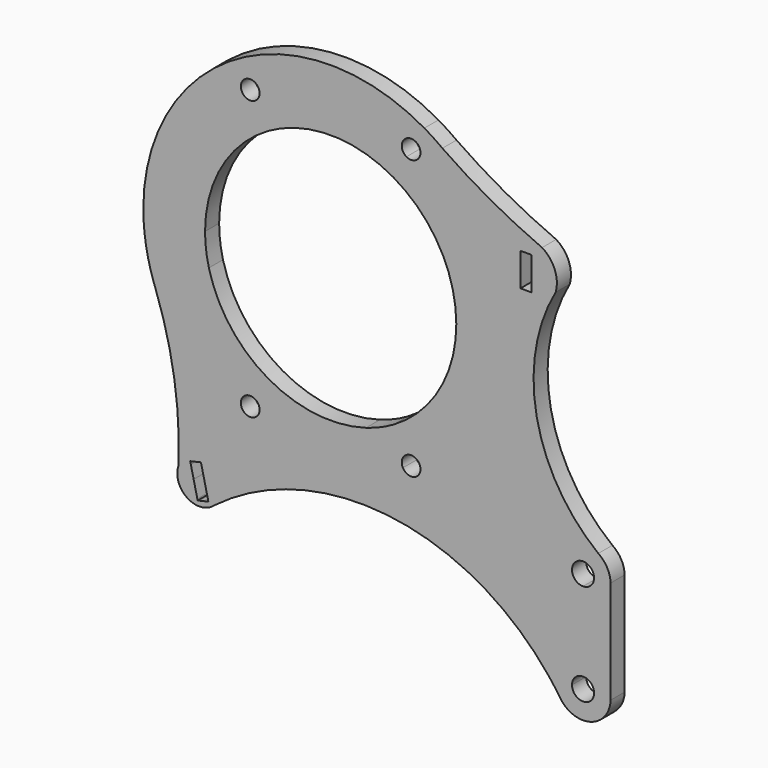
from build123d import *

# Parameters (mm, degrees)
F0_W     = 5
F0_H     = 15
F1_DEPTH = 8


with BuildPart() as f1:
    # F0 (on Front) → F1 (new body)
    with BuildSketch(Plane.XZ):
        with BuildLine():
            ThreePointArc((96.051040545, -74.4952633909), (99.586574451, -75.9597294849), (101.051040545, -79.4952633909))
            Line((101.051040545, -79.4952633909), (108.5446846503, -79.4952633909))
            Line((108.5446846503, -79.4952633909), (108.5446846503, -79.0966947381))
            Line((108.5446846503, -79.0966947381), (108.5446846503, -33.8938320436))
            Line((108.5446846503, -33.8938320436), (108.5446846503, -33.0966947381))
            ThreePointArc((108.5446846503, -33.0966947381), (106.9735378091, -27.4166900782), (102.9745588744, -23.0878192309))
            ThreePointArc((102.9745588744, -23.0878192309), (75.0475031004, 22.3518348869), (83.6459918624, 74.9897356957))
            ThreePointArc((83.6459918624, 74.9897356957), (83.213349074, 83.916829816), (77.4679593625, 90.763046748))
            ThreePointArc((77.4679593625, 90.763046748), (54.2323791008, 102.1278384031), (32.237536797, 115.739509553))
            ThreePointArc((32.237536797, 115.739509553), (46.3985337021, 102.4586914011), (57.1766192186, 86.3110340872))
            ThreePointArc((57.1766192186, 86.3110340872), (64.1749741493, 67.4661239993), (66.5520777255, 47.5047366091))
            ThreePointArc((66.5520777255, 47.5047366091), (55.1642370471, 5.0047366091), (24.0520777255, -26.1074227125))
            ThreePointArc((24.0520777255, -26.1074227125), (11.2153330726, -32.151344654), (-2.4479222745, -35.9758000446))
            Line((-2.4479222745, -35.9758000446), (-2.4479222745, -38.2282986652))
            ThreePointArc((-2.4479222745, -38.2282986652), (43.6638893075, -49.6244865639), (80.5950273587, -79.4952633909))
            Line((80.5950273587, -79.4952633909), (91.051040545, -79.4952633909))
            ThreePointArc((91.051040545, -79.4952633909), (92.5155066391, -75.9597294849), (96.051040545, -74.4952633909))
        make_face()
        with BuildLine():
            ThreePointArc((101.051040545, -33.4952633909), (99.586574451, -37.0307972968), (96.051040545, -38.4952633909))
            ThreePointArc((96.051040545, -38.4952633909), (92.5155066391, -29.9597294849), (101.051040545, -33.4952633909))
        make_face(mode=Mode.SUBTRACT)
        with Locations((70.1775963157, 78.8110340872)):
            Rectangle(F0_W, F0_H, mode=Mode.SUBTRACT)
        with BuildLine():
            Line((108.5446846503, -79.4952633909), (101.051040545, -79.4952633909))
            ThreePointArc((101.051040545, -79.4952633909), (96.051040545, -84.4952633909), (91.051040545, -79.4952633909))
            Line((91.051040545, -79.4952633909), (80.5950273587, -79.4952633909))
            ThreePointArc((80.5950273587, -79.4952633909), (83.0087277773, -82.6464275943), (85.3064858893, -85.8831069432))
            ThreePointArc((85.3064858893, -85.8831069432), (99.1707652013, -91.5996972095), (108.5446846503, -79.8938320436))
            Line((108.5446846503, -79.8938320436), (108.5446846503, -79.4952633909))
        make_face()
        with BuildLine():
            ThreePointArc((-49.4766412308, -47.648732709), (-26.485075504, -40.328623161), (-2.4479222745, -38.2282986652))
            Line((-2.4479222745, -38.2282986652), (-2.4479222745, -35.9758000446))
            ThreePointArc((-2.4479222745, -35.9758000446), (-59.8941418394, -26.7058481061), (-97.9165682257, 17.3429344301))
            ThreePointArc((-97.9165682257, 17.3429344301), (-89.4001229489, -15.7837478144), (-87.5014994409, -49.9349139067))
            ThreePointArc((-87.5014994409, -49.9349139067), (-87.0083312551, -48.7555482085), (-86.3687393855, -47.648732709))
            ThreePointArc((-86.3687393855, -47.648732709), (-82.7667512172, -44.3786510364), (-78.0479222745, -43.1952633909))
            Line((-78.0479222745, -43.1952633909), (-78.0479222745, -42.0817346844))
            Line((-78.0479222745, -42.0817346844), (-77.7900763305, -43.1985881701))
            ThreePointArc((-77.7900763305, -43.1985881701), (-73.2158097389, -44.4402255016), (-69.7271051635, -47.648732709))
            Line((-69.7271051635, -47.648732709), (-49.4766412308, -47.648732709))
        make_face()
        with BuildLine():
            ThreePointArc((-97.9165682257, 17.3429344301), (-59.8941418394, -26.7058481061), (-2.4479222745, -35.9758000446))
            Line((-2.4479222745, -35.9758000446), (-2.4479222745, -23.7202590034))
            ThreePointArc((-2.4479222745, -23.7202590034), (-27.346314823, -24.9508954014), (-51.2070161773, -17.7320763623))
            ThreePointArc((-51.2070161773, -17.7320763623), (-57.0729222745, -19.3957258332), (-58.5651126184, -13.4838774013))
            ThreePointArc((-58.5651126184, -13.4838774013), (-79.0670356762, 6.8313658317), (-90.0928802269, 33.5047366091))
            Line((-90.0928802269, 33.5047366091), (-102.2870539494, 33.5047366091))
            ThreePointArc((-102.2870539494, 33.5047366091), (-100.6924729992, 26.0376949849), (-98.4342508199, 18.7438735165))
            ThreePointArc((-98.4342508199, 18.7438735165), (-98.1739124224, 18.0439571899), (-97.9165682257, 17.3429344301))
        make_face()
        with BuildLine():
            Line((-2.4479222745, -23.7202590034), (-2.4479222745, -35.9758000446))
            ThreePointArc((-2.4479222745, -35.9758000446), (11.2153330726, -32.151344654), (24.0520777255, -26.1074227125))
            Line((24.0520777255, -26.1074227125), (20.1770777255, -19.3957258332))
            ThreePointArc((20.1770777255, -19.3957258332), (16.8924568739, -19.8038559953), (14.3111716282, -17.7320763623))
            ThreePointArc((14.3111716282, -17.7320763623), (6.1147911828, -21.2387947783), (-2.4479222745, -23.7202590034))
        make_face()
        with BuildLine():
            ThreePointArc((-71.1328973462, -60.4558025605), (-60.6742880355, -53.4274258311), (-49.4766412308, -47.648732709))
            Line((-49.4766412308, -47.648732709), (-69.7271051635, -47.648732709))
            ThreePointArc((-69.7271051635, -47.648732709), (-68.4769199469, -50.2976929525), (-68.0479222745, -53.1952633909))
            ThreePointArc((-68.0479222745, -53.1952633909), (-68.8619607706, -57.1472390041), (-71.1715445241, -60.4558025605))
            Line((-71.1715445241, -60.4558025605), (-71.1328973462, -60.4558025605))
        make_face()
        with BuildLine():
            ThreePointArc((-51.2070161773, -17.7320763623), (-27.346314823, -24.9508954014), (-2.4479222745, -23.7202590034))
            Line((-2.4479222745, -23.7202590034), (-2.4479222745, -7.2035808572))
            ThreePointArc((-2.4479222745, -7.2035808572), (-25.2453046649, -9.0885102728), (-46.9479222745, -1.8587114066))
            Line((-46.9479222745, -1.8587114066), (-52.8229222745, -12.034509901))
            ThreePointArc((-52.8229222745, -12.034509901), (-51.2673143085, -13.5901178671), (-50.6979222745, -15.7151178671))
            ThreePointArc((-50.6979222745, -15.7151178671), (-50.8271607604, -16.755225815), (-51.2070161773, -17.7320763623))
        make_face()
        with BuildLine():
            Line((-2.4479222745, -7.2035808572), (-2.4479222745, -23.7202590034))
            ThreePointArc((-2.4479222745, -23.7202590034), (6.1147911828, -21.2387947783), (14.3111716282, -17.7320763623))
            ThreePointArc((14.3111716282, -17.7320763623), (13.9633395973, -14.5554970156), (15.9270777255, -12.034509901))
            Line((15.9270777255, -12.034509901), (10.0520777255, -1.8587114066))
            ThreePointArc((10.0520777255, -1.8587114066), (3.9619953371, -4.9051440684), (-2.4479222745, -7.2035808572))
        make_face()
        with BuildLine():
            Line((20.1770777255, -19.3957258332), (24.0520777255, -26.1074227125))
            ThreePointArc((24.0520777255, -26.1074227125), (55.1642370471, 5.0047366091), (66.5520777255, 47.5047366091))
            ThreePointArc((66.5520777255, 47.5047366091), (64.1749741493, 67.4661239993), (57.1766192186, 86.3110340872))
            ThreePointArc((57.1766192186, 86.3110340872), (46.3985337021, 102.4586914011), (32.237536797, 115.739509553))
            ThreePointArc((32.237536797, 115.739509553), (28.2223200289, 118.5461926988), (24.0520777255, 121.1168959308))
            Line((24.0520777255, 121.1168959308), (20.1770777255, 114.4051990515))
            ThreePointArc((20.1770777255, 114.4051990515), (21.7326856915, 112.8495910854), (22.3020777255, 110.7245910854))
            ThreePointArc((22.3020777255, 110.7245910854), (22.1408158536, 109.5649702339), (21.6692680693, 108.4933506196))
            ThreePointArc((21.6692680693, 108.4933506196), (45.8076412788, 82.1489648795), (54.5520777255, 47.5047366091))
            ThreePointArc((54.5520777255, 47.5047366091), (45.8076412788, 12.8605083388), (21.6692680693, -13.4838774013))
            ThreePointArc((21.6692680693, -13.4838774013), (22.1408158536, -14.5554970156), (22.3020777255, -15.7151178671))
            ThreePointArc((22.3020777255, -15.7151178671), (21.7326856915, -17.8401178671), (20.1770777255, -19.3957258332))
        make_face()
        with BuildLine():
            ThreePointArc((-68.0479222745, -53.1952633909), (-68.4769199469, -50.2976929525), (-69.7271051635, -47.648732709))
            Line((-69.7271051635, -47.648732709), (-76.7626795106, -47.648732709))
            Line((-76.7626795106, -47.648732709), (-75.4821620051, -53.1952633909))
            Line((-75.4821620051, -53.1952633909), (-73.924864205, -59.9406612409))
            Line((-73.924864205, -59.9406612409), (-73.8059344604, -60.4558025605))
            Line((-73.8059344604, -60.4558025605), (-71.1715445241, -60.4558025605))
            ThreePointArc((-71.1715445241, -60.4558025605), (-68.8619607706, -57.1472390041), (-68.0479222745, -53.1952633909))
        make_face()
        with BuildLine():
            Line((-76.7626795106, -47.648732709), (-69.7271051635, -47.648732709))
            ThreePointArc((-69.7271051635, -47.648732709), (-73.2158097389, -44.4402255016), (-77.7900763305, -43.1985881701))
            Line((-77.7900763305, -43.1985881701), (-77.2991300202, -45.3251102691))
            Line((-77.2991300202, -45.3251102691), (-76.7626795106, -47.648732709))
        make_face()
        with BuildLine():
            ThreePointArc((-86.3687393855, -47.648732709), (-87.0083312551, -48.7555482085), (-87.5014994409, -49.9349139067))
            ThreePointArc((-87.5014994409, -49.9349139067), (-87.9103705422, -51.5423525741), (-88.0479222745, -53.1952633909))
            Line((-88.0479222745, -53.1952633909), (-80.613682544, -53.1952633909))
            Line((-80.613682544, -53.1952633909), (-81.8942000496, -47.648732709))
            Line((-81.8942000496, -47.648732709), (-86.3687393855, -47.648732709))
        make_face()
        with BuildLine():
            ThreePointArc((-71.3521437188, -60.6226821573), (-71.2613311641, -60.5397974877), (-71.1715445241, -60.4558025605))
            Line((-71.1715445241, -60.4558025605), (-73.8059344604, -60.4558025605))
            Line((-73.8059344604, -60.4558025605), (-76.1561864026, -60.4558025605))
            Line((-76.1561864026, -60.4558025605), (-78.0479222745, -60.8925441993))
            Line((-78.0479222745, -60.8925441993), (-78.0479222745, -63.1952633909))
            ThreePointArc((-78.0479222745, -63.1952633909), (-74.4614328813, -62.5299885519), (-71.3521437188, -60.6226821573))
        make_face()
        with BuildLine():
            ThreePointArc((-78.0479222745, -43.1952633909), (-77.9189885852, -43.1960946202), (-77.7900763305, -43.1985881701))
            Line((-77.7900763305, -43.1985881701), (-78.0479222745, -42.0817346844))
            Line((-78.0479222745, -42.0817346844), (-78.0479222745, -43.1952633909))
        make_face()
        with BuildLine():
            Line((-77.2991300202, -45.3251102691), (-77.7900763305, -43.1985881701))
            ThreePointArc((-77.7900763305, -43.1985881701), (-77.9189885852, -43.1960946202), (-78.0479222745, -43.1952633909))
            Line((-78.0479222745, -43.1952633909), (-78.0479222745, -45.4979825824))
            Line((-78.0479222745, -45.4979825824), (-77.2991300202, -45.3251102691))
        make_face()
        with BuildLine():
            Line((-52.8229222745, -12.034509901), (-46.9479222745, -1.8587114066))
            ThreePointArc((-46.9479222745, -1.8587114066), (-63.9047675407, 13.1146912697), (-73.7018814087, 33.5047366091))
            Line((-73.7018814087, 33.5047366091), (-90.0928802269, 33.5047366091))
            ThreePointArc((-90.0928802269, 33.5047366091), (-79.0670356762, 6.8313658317), (-58.5651126184, -13.4838774013))
            ThreePointArc((-58.5651126184, -13.4838774013), (-55.9880302224, -11.5943563529), (-52.8229222745, -12.034509901))
        make_face()
        with BuildLine():
            ThreePointArc((38.5520777255, 47.5047366091), (30.9155257412, 19.0047366091), (10.0520777255, -1.8587114066))
            Line((10.0520777255, -1.8587114066), (15.9270777255, -12.034509901))
            ThreePointArc((15.9270777255, -12.034509901), (19.0921856734, -11.5943563529), (21.6692680693, -13.4838774013))
            ThreePointArc((21.6692680693, -13.4838774013), (45.8076412788, 12.8605083388), (54.5520777255, 47.5047366091))
            ThreePointArc((54.5520777255, 47.5047366091), (45.8076412788, 82.1489648795), (21.6692680693, 108.4933506196))
            ThreePointArc((21.6692680693, 108.4933506196), (19.0921856734, 106.6038295712), (15.9270777255, 107.0439831193))
            Line((15.9270777255, 107.0439831193), (10.0520777255, 96.8681846249))
            ThreePointArc((10.0520777255, 96.8681846249), (30.9155257412, 76.0047366091), (38.5520777255, 47.5047366091))
        make_face()
        with BuildLine():
            ThreePointArc((-103.4479222745, 47.5047366091), (-103.1572080476, 40.4807132737), (-102.2870539494, 33.5047366091))
            Line((-102.2870539494, 33.5047366091), (-90.0928802269, 33.5047366091))
            ThreePointArc((-90.0928802269, 33.5047366091), (-91.1083720754, 40.4720248464), (-91.4479222745, 47.5047366091))
            Line((-91.4479222745, 47.5047366091), (-103.4479222745, 47.5047366091))
        make_face()
        with BuildLine():
            ThreePointArc((-78.0479222745, -43.1952633909), (-82.7667512172, -44.3786510364), (-86.3687393855, -47.648732709))
            Line((-86.3687393855, -47.648732709), (-81.8942000496, -47.648732709))
            Line((-81.8942000496, -47.648732709), (-82.1709803441, -46.4498655408))
            Line((-82.1709803441, -46.4498655408), (-78.0479222745, -45.4979825824))
            Line((-78.0479222745, -45.4979825824), (-78.0479222745, -43.1952633909))
        make_face()
        with BuildLine():
            Line((-80.613682544, -53.1952633909), (-88.0479222745, -53.1952633909))
            ThreePointArc((-88.0479222745, -53.1952633909), (-87.2338837785, -57.1472390041), (-84.924300025, -60.4558025605))
            Line((-84.924300025, -60.4558025605), (-78.9374549993, -60.4558025605))
            Line((-78.9374549993, -60.4558025605), (-80.613682544, -53.1952633909))
        make_face()
        Polygon((-76.1561864026, -60.4558025605), (-73.8059344604, -60.4558025605), (-73.924864205, -59.9406612409), align=None)
        with BuildLine():
            ThreePointArc((-84.924300025, -60.4558025605), (-81.7489091905, -62.4851878172), (-78.0479222745, -63.1952633909))
            Line((-78.0479222745, -63.1952633909), (-78.0479222745, -60.8925441993))
            Line((-78.0479222745, -60.8925441993), (-78.7967145289, -61.0654165126))
            Line((-78.7967145289, -61.0654165126), (-78.9374549993, -60.4558025605))
            Line((-78.9374549993, -60.4558025605), (-84.924300025, -60.4558025605))
        make_face()
        with BuildLine():
            Line((-90.0928802269, 33.5047366091), (-73.7018814087, 33.5047366091))
            ThreePointArc((-73.7018814087, 33.5047366091), (-75.0097277206, 40.450506341), (-75.4479222745, 47.5047366091))
            Line((-75.4479222745, 47.5047366091), (-91.4479222745, 47.5047366091))
            ThreePointArc((-91.4479222745, 47.5047366091), (-91.1083720754, 40.4720248464), (-90.0928802269, 33.5047366091))
        make_face()
        with BuildLine():
            ThreePointArc((-60.9479222745, 121.1168959308), (-92.0600815962, 90.0047366091), (-103.4479222745, 47.5047366091))
            Line((-103.4479222745, 47.5047366091), (-91.4479222745, 47.5047366091))
            ThreePointArc((-91.4479222745, 47.5047366091), (-82.7034858278, 82.1489648795), (-58.5651126184, 108.4933506196))
            ThreePointArc((-58.5651126184, 108.4933506196), (-59.0686837887, 111.7646990333), (-57.0729222745, 114.4051990515))
            Line((-57.0729222745, 114.4051990515), (-60.9479222745, 121.1168959308))
        make_face()
        with BuildLine():
            Line((-91.4479222745, 47.5047366091), (-75.4479222745, 47.5047366091))
            ThreePointArc((-75.4479222745, 47.5047366091), (-67.8113702903, 76.0047366091), (-46.9479222745, 96.8681846249))
            Line((-46.9479222745, 96.8681846249), (-52.8229222745, 107.0439831193))
            ThreePointArc((-52.8229222745, 107.0439831193), (-55.9880302224, 106.6038295712), (-58.5651126184, 108.4933506196))
            ThreePointArc((-58.5651126184, 108.4933506196), (-82.7034858278, 82.1489648795), (-91.4479222745, 47.5047366091))
        make_face()
        with BuildLine():
            ThreePointArc((-46.9479222745, 96.8681846249), (-18.4479222745, 104.5047366091), (10.0520777255, 96.8681846249))
            Line((10.0520777255, 96.8681846249), (15.9270777255, 107.0439831193))
            ThreePointArc((15.9270777255, 107.0439831193), (13.9633395973, 109.5649702339), (14.3111716282, 112.7415495806))
            ThreePointArc((14.3111716282, 112.7415495806), (-18.4479222745, 120.5047366091), (-51.2070161773, 112.7415495806))
            ThreePointArc((-51.2070161773, 112.7415495806), (-50.8271607604, 111.7646990333), (-50.6979222745, 110.7245910854))
            ThreePointArc((-50.6979222745, 110.7245910854), (-51.2673143085, 108.5995910854), (-52.8229222745, 107.0439831193))
            Line((-52.8229222745, 107.0439831193), (-46.9479222745, 96.8681846249))
        make_face()
        with BuildLine():
            ThreePointArc((24.0520777255, 121.1168959308), (-18.4479222745, 132.5047366091), (-60.9479222745, 121.1168959308))
            Line((-60.9479222745, 121.1168959308), (-57.0729222745, 114.4051990515))
            ThreePointArc((-57.0729222745, 114.4051990515), (-53.788301423, 114.8133292136), (-51.2070161773, 112.7415495806))
            ThreePointArc((-51.2070161773, 112.7415495806), (-18.4479222745, 120.5047366091), (14.3111716282, 112.7415495806))
            ThreePointArc((14.3111716282, 112.7415495806), (16.8924568739, 114.8133292136), (20.1770777255, 114.4051990515))
            Line((20.1770777255, 114.4051990515), (24.0520777255, 121.1168959308))
        make_face()
    extrude(amount=F1_DEPTH)


solid = f1.part
